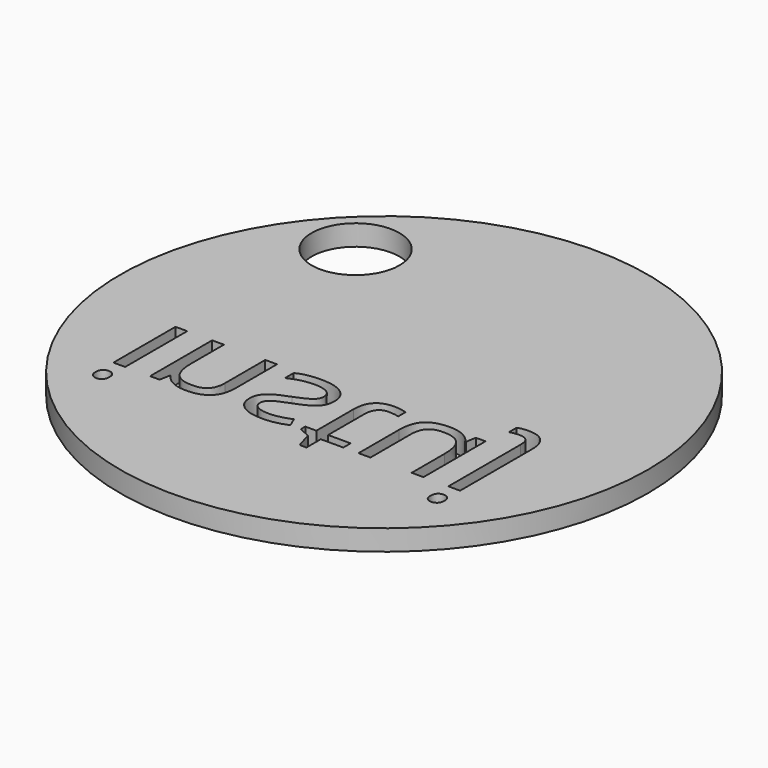
from build123d import *

# Parameters (mm, degrees)
F0_R         = 27.4
F1_DEPTH     = 2.15
F4_R         = 4.5563821827
F5_DEPTH     = 2.15
F6_TEXT_SIZE = 15.0488747749
F7_DEPTH     = 2.15


# Not quite as in the source:
# - Text() gives the source's letters only with a copy of the font that has no kerning and outlines rounded to 1/6400 em; it was checked with that copy


with BuildPart() as f1:
    # F0 (on Top) → F1 (new body)
    with BuildSketch(Plane.XY):
        Circle(F0_R)
    extrude(amount=F1_DEPTH)

    # F4 (on face) → F5 (cut, through all)
    with BuildSketch(Plane.XY.offset(2.15)):
        with Locations((-15.2985882014, 15.4223609716)):
            Circle(F4_R)
    extrude(amount=-F5_DEPTH, mode=Mode.SUBTRACT)

    # F6 (on face) → F7 (cut, through all)
    with BuildSketch(Plane(origin=(0, 0, 0), x_dir=(1, 0, 0), z_dir=(0, 0, -1))):
        with Locations((-19.4784917403, 4.3375599198)):
            Text('instuj', F6_TEXT_SIZE, font='Open Sans', text_align=(TextAlign.LEFT, TextAlign.BOTTOM))
    extrude(amount=-F7_DEPTH, mode=Mode.SUBTRACT)


solid = f1.part
